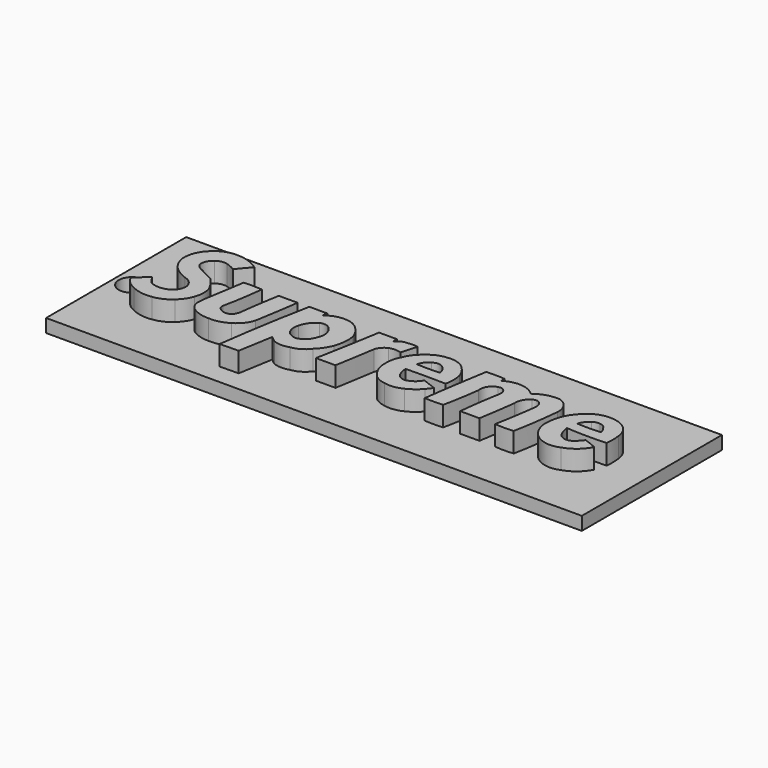
from build123d import *

# Parameters (mm, degrees)
F1_W     = 80.755950883
F1_H     = 26.4027640224
F1_R     = 2
F2_DEPTH = 2
F3_DEPTH = 5


with BuildPart() as f2:
    # F1 (on Top) → F2 (new body)
    with BuildSketch(Plane.XY):
        with Locations((-8.9335693046, 13.2013820112)):
            Rectangle(F1_W, F1_H)
        with Locations((-46.6689318419, 12.8928329796)):
            Circle(F1_R, mode=Mode.SUBTRACT)
    extrude(amount=F2_DEPTH)


with BuildPart() as f3:
    # F0 (on Top) → F3 (new body)
    with BuildSketch(Plane.XY):
        with BuildLine():
            ThreePointArc((-36.2984538078, 18.9516562968), (-35.4830710925, 19.9453504297), (-34.6325263381, 20.9091193974))
            ThreePointArc((-34.6325263381, 20.9091193974), (-36.3668311326, 21.800866294), (-38.2975637913, 22.0752693713))
            ThreePointArc((-38.2975637913, 22.0752693713), (-39.898509652, 21.7711277671), (-41.2545837462, 20.8674725145))
            ThreePointArc((-41.2545837462, 20.8674725145), (-42.3456459486, 19.3415051227), (-42.670622468, 17.4939706922))
            ThreePointArc((-42.670622468, 17.4939706922), (-42.2161284241, 16.0265436075), (-41.2545837462, 14.8284872994))
            ThreePointArc((-41.2545837462, 14.8284872994), (-40.3396754086, 14.2109845283), (-39.3387675285, 13.7456348166))
            ThreePointArc((-39.3387675285, 13.7456348166), (-38.3635703507, 13.1945790167), (-37.839435041, 12.2046526521))
            ThreePointArc((-37.839435041, 12.2046526521), (-38.087109557, 11.0281471625), (-38.9639362693, 10.2055398747))
            ThreePointArc((-38.9639362693, 10.2055398747), (-40.2550287545, 9.9213273636), (-41.5461212397, 10.2055398747))
            ThreePointArc((-41.5461212397, 10.2055398747), (-42.0283685065, 10.7911428797), (-42.4623824656, 11.4133367315))
            ThreePointArc((-42.4623824656, 11.4133367315), (-43.4193369359, 10.620866872), (-44.3781986833, 9.8307058215))
            ThreePointArc((-44.3781986833, 9.8307058215), (-43.6032075218, 8.7232146174), (-42.4623824656, 7.9981861636))
            ThreePointArc((-42.4623824656, 7.9981861636), (-40.9422867039, 7.4875987817), (-39.3387675285, 7.4984086677))
            ThreePointArc((-39.3387675285, 7.4984086677), (-37.9946192046, 7.8785450642), (-36.8398800492, 8.6645577103))
            ThreePointArc((-36.8398800492, 8.6645577103), (-36.0033516186, 9.5843664901), (-35.465490073, 10.7053183019))
            ThreePointArc((-35.465490073, 10.7053183019), (-35.2099262734, 12.0797078125), (-35.465490073, 13.4540973231))
            ThreePointArc((-35.465490073, 13.4540973231), (-36.0913584305, 14.4560006261), (-36.8398800492, 15.3699135408))
            ThreePointArc((-36.8398800492, 15.3699135408), (-37.9124468802, 15.9122572154), (-38.9639362693, 16.4944138378))
            ThreePointArc((-38.9639362693, 16.4944138378), (-39.6245277455, 16.8538860262), (-40.1300862432, 17.4106732011))
            ThreePointArc((-40.1300862432, 17.4106732011), (-39.995082428, 18.4394897255), (-39.3387675285, 19.2431937903))
            ThreePointArc((-39.3387675285, 19.2431937903), (-38.5445904431, 19.6037101293), (-37.6728437841, 19.5763781667))
            ThreePointArc((-37.6728437841, 19.5763781667), (-36.9644492284, 19.3106563436), (-36.2984538078, 18.9516562968))
        make_face()
    extrude(amount=F3_DEPTH)


with BuildPart() as f3b:
    # F0 (on Top) → F3, piece 2 (new body)
    with BuildSketch(Plane.XY):
        with BuildLine():
            ThreePointArc((-31.3839688897, 10.9552070498), (-30.826132377, 13.9830968737), (-30.4260607809, 17.0358400792))
            ThreePointArc((-30.4260607809, 17.0358400792), (-31.7997996894, 17.0995728468), (-33.1748388708, 17.0774888247))
            ThreePointArc((-33.1748388708, 17.0774888247), (-33.6132760709, 14.3214926657), (-34.061819315, 11.5671232343))
            ThreePointArc((-34.061819315, 11.5671232343), (-34.1945619623, 10.6427534641), (-34.2679694295, 9.7117908299))
            ThreePointArc((-34.2679694295, 9.7117908299), (-33.9012849934, 8.6923059284), (-33.0899804831, 7.974258624))
            ThreePointArc((-33.0899804831, 7.974258624), (-31.9656063493, 7.5175442373), (-30.7592451572, 7.3852646165))
            ThreePointArc((-30.7592451572, 7.3852646165), (-29.2426695896, 7.5201936412), (-27.8438739479, 8.1215072423))
            ThreePointArc((-27.8438739479, 8.1215072423), (-26.7186419602, 9.0913253851), (-26.0515008122, 10.4185845703))
            ThreePointArc((-26.0515008122, 10.4185845703), (-25.504221846, 13.7226115832), (-25.0157285482, 17.0358400792))
            ThreePointArc((-25.0157285482, 17.0358400792), (-26.429801248, 17.0151497516), (-27.8438739479, 17.0358400792))
            ThreePointArc((-27.8438739479, 17.0358400792), (-28.3488737079, 14.0025861759), (-28.7601333112, 10.9552070498))
            ThreePointArc((-28.7601333112, 10.9552070498), (-28.925916607, 10.4067605969), (-29.2182639241, 9.9140023813))
            ThreePointArc((-29.2182639241, 9.9140023813), (-29.9887545407, 9.6923938605), (-30.7592451572, 9.9140023813))
            ThreePointArc((-30.7592451572, 9.9140023813), (-31.2548604383, 10.3246525028), (-31.3839688897, 10.9552070498))
        make_face()
    extrude(amount=F3_DEPTH)


with BuildPart() as f3c:
    # F0 (on Top) → F3, piece 3 (new body)
    with BuildSketch(Plane.XY):
        with BuildLine():
            ThreePointArc((-20.676124841, 16.3217391819), (-20.6354540742, 16.7065480767), (-20.5252952874, 17.0774888247))
            ThreePointArc((-20.5252952874, 17.0774888247), (-21.908656694, 17.0789249817), (-23.2920181006, 17.0774888247))
            ThreePointArc((-23.2920181006, 17.0774888247), (-24.5671501441, 10.0977370451), (-25.6081279367, 3.0792427715))
            ThreePointArc((-25.6081279367, 3.0792427715), (-24.1985227187, 3.1105454566), (-22.7886710389, 3.1274265042))
            ThreePointArc((-22.7886710389, 3.1274265042), (-22.341671656, 5.7540784164), (-21.8952819705, 8.3808340132))
            ThreePointArc((-21.8952819705, 8.3808340132), (-21.4465474953, 7.9686372868), (-20.9496933967, 7.6159266755))
            ThreePointArc((-20.9496933967, 7.6159266755), (-19.7864295915, 7.4163881202), (-18.6231657863, 7.6159266755))
            ThreePointArc((-18.6231657863, 7.6159266755), (-17.2967272064, 8.0553130605), (-16.267189756, 9.0000629425))
            ThreePointArc((-16.267189756, 9.0000629425), (-15.413918604, 9.99868852), (-14.8156350479, 11.1680394039))
            ThreePointArc((-14.8156350479, 11.1680394039), (-14.4722769179, 12.72527078), (-14.5211378112, 14.3191581592))
            ThreePointArc((-14.5211378112, 14.3191581592), (-15.0278394589, 15.4004202934), (-15.7874748111, 16.3217391819))
            ThreePointArc((-15.7874748111, 16.3217391819), (-16.8838002932, 17.0300611336), (-18.1729011238, 17.2346793115))
            ThreePointArc((-18.1729011238, 17.2346793115), (-19.5080719209, 17.0073225367), (-20.676124841, 16.3217391819))
        make_face()
        with BuildLine():
            ThreePointArc((-18.5869764537, 14.6166225895), (-17.5500284718, 13.2499434504), (-17.7127812058, 11.5421423689))
            ThreePointArc((-17.7127812058, 11.5421423689), (-18.3727628252, 10.4675682896), (-19.477667287, 9.8597267643))
            ThreePointArc((-19.477667287, 9.8597267643), (-20.30476789, 10.0323748319), (-20.9951400757, 10.5194980279))
            ThreePointArc((-20.9951400757, 10.5194980279), (-21.3801551069, 11.4907454057), (-21.2920363992, 12.5317992643))
            ThreePointArc((-21.2920363992, 12.5317992643), (-20.7624961245, 13.7354459261), (-19.7864295915, 14.6166225895))
            ThreePointArc((-19.7864295915, 14.6166225895), (-19.1867030226, 14.7391988845), (-18.5869764537, 14.6166225895))
        make_face(mode=Mode.SUBTRACT)
    extrude(amount=F3_DEPTH)


with BuildPart() as f3d:
    # F0 (on Top) → F3, piece 4 (new body)
    with BuildSketch(Plane.XY):
        with BuildLine():
            ThreePointArc((-10.0679956377, 17.0774888247), (-11.4215617068, 17.0705631875), (-12.775127776, 17.0774888247))
            ThreePointArc((-12.775127776, 17.0774888247), (-13.6136939234, 12.2135104729), (-14.5211378112, 7.3619103059))
            ThreePointArc((-14.5211378112, 7.3619103059), (-13.0498996004, 7.3614335223), (-11.5786613896, 7.3619103059))
            ThreePointArc((-11.5786613896, 7.3619103059), (-11.0725779535, 10.3730049912), (-10.5885975063, 13.3877312765))
            ThreePointArc((-10.5885975063, 13.3877312765), (-10.1711725419, 14.1567677772), (-9.4849206507, 14.6996481344))
            ThreePointArc((-9.4849206507, 14.6996481344), (-8.558249101, 14.8500262213), (-7.6315775514, 14.6996481344))
            ThreePointArc((-7.6315775514, 14.6996481344), (-7.3118130722, 15.8923296261), (-6.9652064703, 17.0774888247))
            ThreePointArc((-6.9652064703, 17.0774888247), (-7.7461099718, 17.1474561973), (-8.5270134732, 17.0774888247))
            ThreePointArc((-8.5270134732, 17.0774888247), (-9.3861616125, 16.8803867566), (-10.0679956377, 16.3217391819))
            ThreePointArc((-10.0679956377, 16.3217391819), (-10.09795242, 16.6996140033), (-10.0679956377, 17.0774888247))
        make_face()
    extrude(amount=F3_DEPTH)


with BuildPart() as f3e:
    # F0 (on Top) → F3, piece 5 (new body)
    with BuildSketch(Plane.XY):
        with BuildLine():
            ThreePointArc((-0.9764094139, 10.8815506101), (-1.6906978752, 10.0438460904), (-2.6749665849, 9.5507213846))
            ThreePointArc((-2.6749665849, 9.5507213846), (-3.6632190893, 9.7407930279), (-4.2859693058, 10.5313323438))
            ThreePointArc((-4.2859693058, 10.5313323438), (-4.4699743419, 11.1507509793), (-4.5486330055, 11.7921167985))
            ThreePointArc((-4.5486330055, 11.7921167985), (-1.5367581509, 11.8343300575), (1.4751167037, 11.7921167985))
            ThreePointArc((1.4751167037, 11.7921167985), (1.6178844678, 13.096679002), (1.4751167037, 14.4012412056))
            ThreePointArc((1.4751167037, 14.4012412056), (0.8920195199, 15.5681863768), (0, 16.5200605989))
            ThreePointArc((0, 16.5200605989), (-1.1567624701, 17.0550442713), (-2.4298140779, 17.1154309064))
            ThreePointArc((-2.4298140779, 17.1154309064), (-3.7799296978, 16.8294011068), (-4.9513834529, 16.0997975618))
            ThreePointArc((-4.9513834529, 16.0997975618), (-6.0285495738, 15.1103568495), (-6.7550064996, 13.8408923522))
            ThreePointArc((-6.7550064996, 13.8408923522), (-7.1872865685, 12.7672758637), (-7.3153548874, 11.6170076653))
            ThreePointArc((-7.3153548874, 11.6170076653), (-7.1873000678, 10.2733383196), (-6.6324300133, 9.0429056436))
            ThreePointArc((-6.6324300133, 9.0429056436), (-5.6497658212, 7.9449210564), (-4.2684581131, 7.431902457))
            ThreePointArc((-4.2684581131, 7.431902457), (-2.8450221264, 7.3580202383), (-1.4842253877, 7.7821202576))
            ThreePointArc((-1.4842253877, 7.7821202576), (-0.4558379774, 8.4010848518), (0.406952051, 9.2355255038))
            ThreePointArc((0.406952051, 9.2355255038), (0.7646954369, 9.6542702488), (1.0723661399, 10.1110702381))
            ThreePointArc((1.0723661399, 10.1110702381), (0.0492296479, 10.4996377013), (-0.9764094139, 10.8815506101))
        make_face()
        with BuildLine():
            ThreePointArc((-0.7662783028, 13.5782286525), (-2.5079600157, 13.4957608279), (-4.250947386, 13.5432071984))
            ThreePointArc((-4.250947386, 13.5432071984), (-3.8703064335, 14.3853615136), (-3.1477608718, 14.9615900591))
            ThreePointArc((-3.1477608718, 14.9615900591), (-2.3772813147, 15.2337901631), (-1.6068017576, 14.9615900591))
            ThreePointArc((-1.6068017576, 14.9615900591), (-1.0607303081, 14.3463507122), (-0.7662783028, 13.5782286525))
        make_face(mode=Mode.SUBTRACT)
    extrude(amount=F3_DEPTH)


with BuildPart() as f3f:
    # F0 (on Top) → F3, piece 6 (new body)
    with BuildSketch(Plane.XY):
        with BuildLine():
            ThreePointArc((6.1077964492, 16.473794356), (6.1131423027, 16.7847499251), (6.1077964492, 17.0957054943))
            ThreePointArc((6.1077964492, 17.0957054943), (4.7228663927, 17.1616174695), (3.3367597498, 17.1286929399))
            ThreePointArc((3.3367597498, 17.1286929399), (2.5515141093, 12.2694429432), (1.8522748724, 7.397073321))
            ThreePointArc((1.8522748724, 7.397073321), (3.2377934549, 7.3516245836), (4.6233120374, 7.397073321))
            ThreePointArc((4.6233120374, 7.397073321), (5.1420125351, 10.1586341704), (5.5469917133, 12.9391485825))
            ThreePointArc((5.5469917133, 12.9391485825), (5.801460144, 14.2063662901), (6.8335449323, 14.9844381958))
            ThreePointArc((6.8335449323, 14.9844381958), (7.3972962281, 15.0165770277), (7.8561902046, 14.6875409409))
            ThreePointArc((7.8561902046, 14.6875409409), (8.0700086735, 14.2466238213), (8.0951759592, 13.7572437525))
            ThreePointArc((8.0951759592, 13.7572437525), (7.5728049156, 10.5869227034), (7.1872300468, 7.397073321))
            ThreePointArc((7.1872300468, 7.397073321), (8.6387472693, 7.4057968373), (10.0902644917, 7.397073321))
            ThreePointArc((10.0902644917, 7.397073321), (10.5229009491, 10.1650311176), (10.914100334, 12.9391485825))
            ThreePointArc((10.914100334, 12.9391485825), (11.1293936706, 14.1087598913), (11.9340857491, 14.9844381958))
            ThreePointArc((11.9340857491, 14.9844381958), (12.463693507, 15.1573053116), (12.9933012649, 14.9844381958))
            ThreePointArc((12.9933012649, 14.9844381958), (13.3836910439, 14.4297669323), (13.4718781337, 13.7572437525))
            ThreePointArc((13.4718781337, 13.7572437525), (13.0162404092, 10.5694777408), (12.463693507, 7.397073321))
            ThreePointArc((12.463693507, 7.397073321), (13.857814949, 7.3240930725), (15.251936391, 7.397073321))
            ThreePointArc((15.251936391, 7.397073321), (15.8577006013, 10.8852105459), (16.2719227374, 14.4012412056))
            ThreePointArc((16.2719227374, 14.4012412056), (15.840407015, 16.063772614), (14.4673334435, 17.0957054943))
            ThreePointArc((14.4673334435, 17.0957054943), (12.5935359069, 16.9143603158), (10.914100334, 16.063772614))
            ThreePointArc((10.914100334, 16.063772614), (9.6105458884, 16.8690465475), (8.0951759592, 17.0957054943))
            ThreePointArc((8.0951759592, 17.0957054943), (7.0712552994, 16.8813558179), (6.1077964492, 16.473794356))
        make_face()
    extrude(amount=F3_DEPTH)


with BuildPart() as f3g:
    # F0 (on Top) → F3, piece 7 (new body)
    with BuildSketch(Plane.XY):
        with BuildLine():
            ThreePointArc((20.1727747917, 10.2727375925), (19.853256688, 11.055515436), (19.6734573692, 11.8816541508))
            ThreePointArc((19.6734573692, 11.8816541508), (22.696226616, 11.7574517542), (25.7207658142, 11.8261743337))
            ThreePointArc((25.7207658142, 11.8261743337), (25.783298377, 12.9669275272), (25.7038902491, 14.1066303477))
            ThreePointArc((25.7038902491, 14.1066303477), (24.7858683817, 16.0803312524), (22.8364728391, 17.048895359))
            ThreePointArc((22.8364728391, 17.048895359), (20.9432006107, 17.0191412629), (19.2627124488, 16.1466021091))
            ThreePointArc((19.2627124488, 16.1466021091), (17.6881711473, 14.2990621262), (17.0000493526, 11.9711719453))
            ThreePointArc((17.0000493526, 11.9711719453), (17.1673205718, 10.0053052858), (18.2130243629, 8.3322497085))
            ThreePointArc((18.2130243629, 8.3322497085), (20.114791437, 7.3320727112), (22.2484953701, 7.5858039781))
            ThreePointArc((22.2484953701, 7.5858039781), (23.9952238462, 8.5445859292), (25.2342764288, 10.1050576195))
            ThreePointArc((25.2342764288, 10.1050576195), (24.2793930516, 10.5211469717), (23.2983119786, 10.8710220084))
            ThreePointArc((23.2983119786, 10.8710220084), (23.1262688999, 10.5264307343), (22.8364728391, 10.2727375925))
            ThreePointArc((22.8364728391, 10.2727375925), (22.3012921814, 9.7589016612), (21.5994026512, 9.5184920356))
            ThreePointArc((21.5994026512, 9.5184920356), (20.7761659611, 9.6876999368), (20.1727747917, 10.2727375925))
        make_face()
        with BuildLine():
            ThreePointArc((19.9566651136, 13.5377924889), (20.3338367343, 14.3224896771), (20.9570340812, 14.9304643273))
            ThreePointArc((20.9570340812, 14.9304643273), (21.4820493079, 15.162243455), (22.0554806292, 15.1854613796))
            ThreePointArc((22.0554806292, 15.1854613796), (22.5915830152, 15.0228319983), (22.9773912579, 14.6166225895))
            ThreePointArc((22.9773912579, 14.6166225895), (23.3142228574, 14.112566619), (23.5069990158, 13.5377924889))
            ThreePointArc((23.5069990158, 13.5377924889), (21.7318320647, 13.476297203), (19.9566651136, 13.5377924889))
        make_face(mode=Mode.SUBTRACT)
    extrude(amount=F3_DEPTH)


solid = Compound([f2.part, f3.part, f3b.part, f3c.part, f3d.part, f3e.part, f3f.part, f3g.part])
